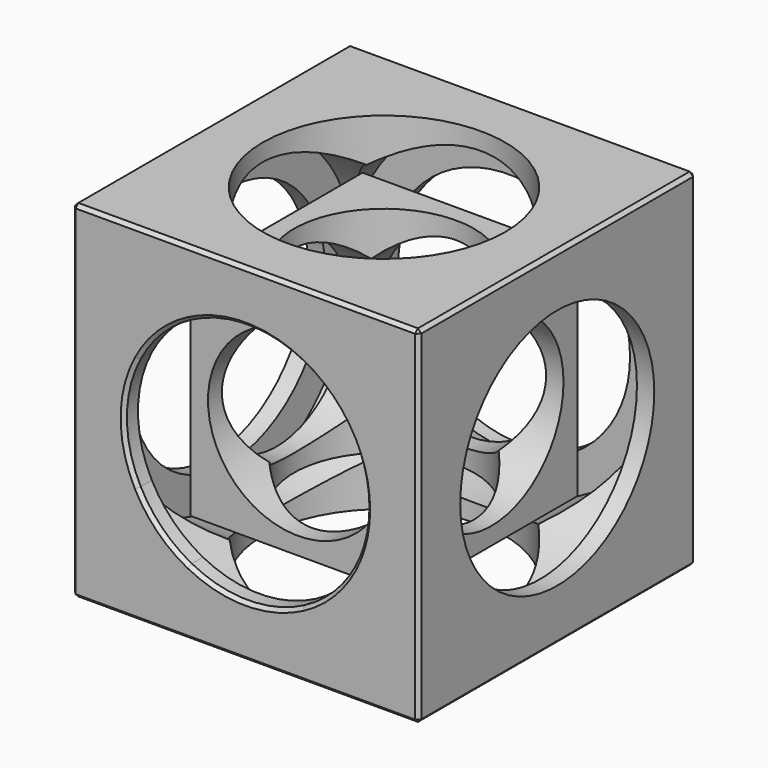
from build123d import *

# Parameters (mm, degrees)
F0_W      = 50
F0_H      = 50
F0_R      = 22.5
F1_DEPTH  = 25
F2_SIZE   = 0.5
F3_R      = 17.5
F4_DEPTH  = 25
F5_R      = 17.5
F6_DEPTH  = 25
F7_DEPTH  = 22.5
F5_R_2    = 22.5
F8_DEPTH  = 22.5
F0_R_2    = 13
F9_DEPTH  = 15.5
F10_R     = 13
F11_DEPTH = 15.5
F12_R     = 13
F13_DEPTH = 15.5


# Not quite as in the source:
# - a feature names something its author has since deleted; it is built from what else it names


with BuildPart() as f1:
    # F0 (on Front) → F1 (new body, symmetric)
    with BuildSketch(Plane.XZ):
        Rectangle(F0_W, F0_H)
        Circle(F0_R, mode=Mode.SUBTRACT)
        Circle(F0_R)
        with BuildLine():
            ThreePointArc((15.5, 8.1240384046), (16.992645468, 4.1833001327), (17.5, 0))
            ThreePointArc((17.5, 0), (16.992645468, -4.1833001327), (15.5, -8.1240384046))
            Line((15.5, -8.1240384046), (15.5, -15.5))
            Line((15.5, -15.5), (8.1240384046, -15.5))
            ThreePointArc((8.1240384046, -15.5), (0, -17.5), (-8.1240384046, -15.5))
            Line((-8.1240384046, -15.5), (-15.5, -15.5))
            Line((-15.5, -15.5), (-15.5, -8.1240384046))
            ThreePointArc((-15.5, -8.1240384046), (-17.5, 0), (-15.5, 8.1240384046))
            Line((-15.5, 8.1240384046), (-15.5, 15.5))
            Line((-15.5, 15.5), (-8.1240384046, 15.5))
            ThreePointArc((-8.1240384046, 15.5), (0, 17.5), (8.1240384046, 15.5))
            Line((8.1240384046, 15.5), (15.5, 15.5))
            Line((15.5, 15.5), (15.5, 8.1240384046))
        make_face(mode=Mode.SUBTRACT)
        with BuildLine():
            ThreePointArc((8.1240384046, 15.5), (12.3743686708, 12.3743686708), (15.5, 8.1240384046))
            Line((15.5, 8.1240384046), (15.5, 15.5))
            Line((15.5, 15.5), (8.1240384046, 15.5))
        make_face()
        with BuildLine():
            Line((15.5, -15.5), (15.5, -8.1240384046))
            ThreePointArc((15.5, -8.1240384046), (12.3743686708, -12.3743686708), (8.1240384046, -15.5))
            Line((8.1240384046, -15.5), (15.5, -15.5))
        make_face()
        with BuildLine():
            Line((-15.5, -15.5), (-8.1240384046, -15.5))
            ThreePointArc((-8.1240384046, -15.5), (-12.3743686708, -12.3743686708), (-15.5, -8.1240384046))
            Line((-15.5, -8.1240384046), (-15.5, -15.5))
        make_face()
        with BuildLine():
            ThreePointArc((-15.5, 8.1240384046), (-12.3743686708, 12.3743686708), (-8.1240384046, 15.5))
            Line((-8.1240384046, 15.5), (-15.5, 15.5))
            Line((-15.5, 15.5), (-15.5, 8.1240384046))
        make_face()
    extrude(amount=F1_DEPTH, both=True)

    # F2
    f2_edges = [f1.edges().sort_by_distance(p)[0] for p in [
        (0, -25, -25),
        (25, -25, 0),
        (0, -25, 25),
        (-25, -25, 0),
        (15.5, -25, -8.124038),
        (25, 0, 25),
        (0, 25, 25),
        (-25, 0, 25),
        (0, 25, -25),
        (25, 25, 0),
        (-25, 25, 0),
        (15.5, 25, -8.124038),
        (25, 0, -25),
        (-25, 0, -25),
    ]]
    chamfer(f2_edges, length=F2_SIZE)

    # F3 (on Top) → F4 (cut, symmetric)
    with BuildSketch(Plane.XY):
        Circle(F3_R)
    extrude(amount=F4_DEPTH, both=True, mode=Mode.SUBTRACT)

    # F5 (on Right) → F6 (cut, symmetric)
    with BuildSketch(Plane.YZ):
        Circle(F5_R)
    extrude(amount=F6_DEPTH, both=True, mode=Mode.SUBTRACT)

    # F0 (on Front) → F7 (cut, symmetric)
    with BuildSketch(Plane.XZ):
        Circle(F0_R)
        with BuildLine():
            ThreePointArc((15.5, 8.1240384046), (16.992645468, 4.1833001327), (17.5, 0))
            ThreePointArc((17.5, 0), (16.992645468, -4.1833001327), (15.5, -8.1240384046))
            Line((15.5, -8.1240384046), (15.5, -15.5))
            Line((15.5, -15.5), (8.1240384046, -15.5))
            ThreePointArc((8.1240384046, -15.5), (0, -17.5), (-8.1240384046, -15.5))
            Line((-8.1240384046, -15.5), (-15.5, -15.5))
            Line((-15.5, -15.5), (-15.5, -8.1240384046))
            ThreePointArc((-15.5, -8.1240384046), (-17.5, 0), (-15.5, 8.1240384046))
            Line((-15.5, 8.1240384046), (-15.5, 15.5))
            Line((-15.5, 15.5), (-8.1240384046, 15.5))
            ThreePointArc((-8.1240384046, 15.5), (0, 17.5), (8.1240384046, 15.5))
            Line((8.1240384046, 15.5), (15.5, 15.5))
            Line((15.5, 15.5), (15.5, 8.1240384046))
        make_face(mode=Mode.SUBTRACT)
        with BuildLine():
            ThreePointArc((8.1240384046, 15.5), (12.3743686708, 12.3743686708), (15.5, 8.1240384046))
            Line((15.5, 8.1240384046), (15.5, 15.5))
            Line((15.5, 15.5), (8.1240384046, 15.5))
        make_face()
        with BuildLine():
            Line((15.5, -15.5), (15.5, -8.1240384046))
            ThreePointArc((15.5, -8.1240384046), (12.3743686708, -12.3743686708), (8.1240384046, -15.5))
            Line((8.1240384046, -15.5), (15.5, -15.5))
        make_face()
        with BuildLine():
            Line((-15.5, -15.5), (-8.1240384046, -15.5))
            ThreePointArc((-8.1240384046, -15.5), (-12.3743686708, -12.3743686708), (-15.5, -8.1240384046))
            Line((-15.5, -8.1240384046), (-15.5, -15.5))
        make_face()
        with BuildLine():
            ThreePointArc((-15.5, 8.1240384046), (-12.3743686708, 12.3743686708), (-8.1240384046, 15.5))
            Line((-8.1240384046, 15.5), (-15.5, 15.5))
            Line((-15.5, 15.5), (-15.5, 8.1240384046))
        make_face()
    extrude(amount=F7_DEPTH, both=True, mode=Mode.SUBTRACT)

    # F5 (on Right) → F8 (cut, symmetric)
    with BuildSketch(Plane.YZ):
        Circle(F5_R_2)
        Circle(F5_R, mode=Mode.SUBTRACT)
    extrude(amount=F8_DEPTH, both=True, mode=Mode.SUBTRACT)


with BuildPart() as f9:
    # F0 (on Front) → F9 (new body, symmetric)
    with BuildSketch(Plane.XZ):
        with BuildLine():
            ThreePointArc((-15.5, 8.1240384046), (-12.3743686708, 12.3743686708), (-8.1240384046, 15.5))
            Line((-8.1240384046, 15.5), (-15.5, 15.5))
            Line((-15.5, 15.5), (-15.5, 8.1240384046))
        make_face()
        with BuildLine():
            Line((15.5, -8.1240384046), (15.5, 8.1240384046))
            ThreePointArc((15.5, 8.1240384046), (12.3743686708, 12.3743686708), (8.1240384046, 15.5))
            Line((8.1240384046, 15.5), (-8.1240384046, 15.5))
            ThreePointArc((-8.1240384046, 15.5), (-12.3743686708, 12.3743686708), (-15.5, 8.1240384046))
            Line((-15.5, 8.1240384046), (-15.5, -8.1240384046))
            ThreePointArc((-15.5, -8.1240384046), (-12.3743686708, -12.3743686708), (-8.1240384046, -15.5))
            Line((-8.1240384046, -15.5), (8.1240384046, -15.5))
            ThreePointArc((8.1240384046, -15.5), (12.3743686708, -12.3743686708), (15.5, -8.1240384046))
        make_face()
        Circle(F0_R_2, mode=Mode.SUBTRACT)
        with BuildLine():
            Line((-15.5, -15.5), (-8.1240384046, -15.5))
            ThreePointArc((-8.1240384046, -15.5), (-12.3743686708, -12.3743686708), (-15.5, -8.1240384046))
            Line((-15.5, -8.1240384046), (-15.5, -15.5))
        make_face()
        with BuildLine():
            Line((15.5, -15.5), (15.5, -8.1240384046))
            ThreePointArc((15.5, -8.1240384046), (12.3743686708, -12.3743686708), (8.1240384046, -15.5))
            Line((8.1240384046, -15.5), (15.5, -15.5))
        make_face()
        with BuildLine():
            ThreePointArc((8.1240384046, 15.5), (12.3743686708, 12.3743686708), (15.5, 8.1240384046))
            Line((15.5, 8.1240384046), (15.5, 15.5))
            Line((15.5, 15.5), (8.1240384046, 15.5))
        make_face()
    extrude(amount=F9_DEPTH, both=True)

    # F10 (on Right) → F11 (cut, symmetric)
    with BuildSketch(Plane.YZ):
        Circle(F10_R)
    extrude(amount=F11_DEPTH, both=True, mode=Mode.SUBTRACT)

    # F12 (on Top) → F13 (cut, symmetric)
    with BuildSketch(Plane.XY):
        Circle(F12_R)
    extrude(amount=F13_DEPTH, both=True, mode=Mode.SUBTRACT)


solid = Compound([f1.part, f9.part])
